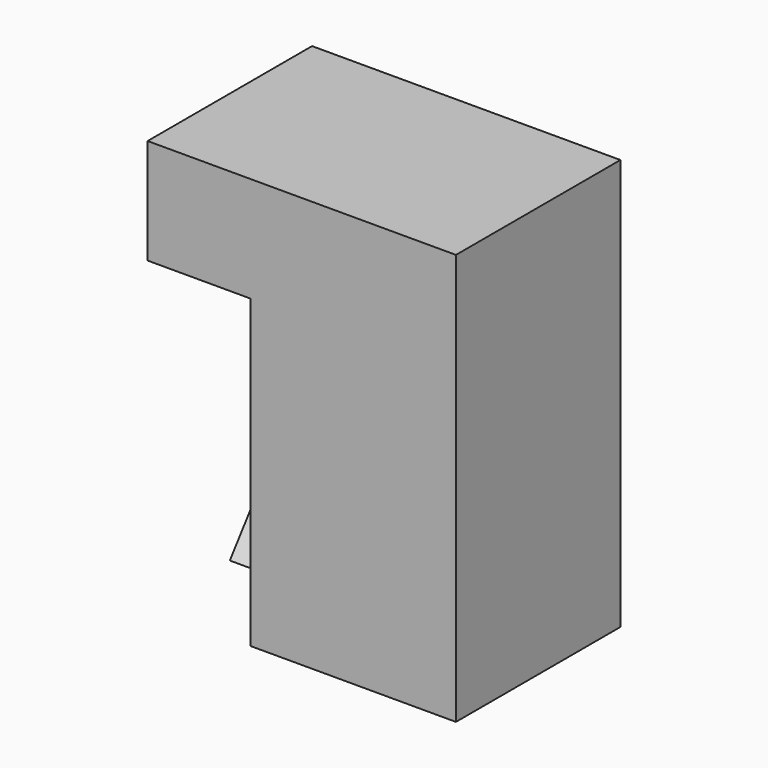
from build123d import *

# Parameters (mm, degrees)
F0_W     = 38.1
F0_H     = 50.8
F1_DEPTH = 25.4
F3_DEPTH = 12.7


# Not quite as in the source:
# - a length typed as a fraction of an inch, garbled in the dataset ("3 / 203.2 mm" for 3/8 in), is restored


with BuildPart() as f1:
    # F0 (on Front) → F1 (new body)
    with BuildSketch(Plane.XZ):
        with Locations((19.05, 25.4)):
            Rectangle(F0_W, F0_H)
    extrude(amount=F1_DEPTH)

    # F2 (on face) → F3 (cut)
    with BuildSketch(Plane(origin=(0, 0, 0), x_dir=(0, -1, 0), z_dir=(-1, 0, 0))):
        Polygon((25.4, 0), (25.4, 37.7936698496), (0, 46.8400232494), (0, 16.886530444), (12.7, 0), align=None)
    extrude(amount=-F3_DEPTH, mode=Mode.SUBTRACT)


solid = f1.part
